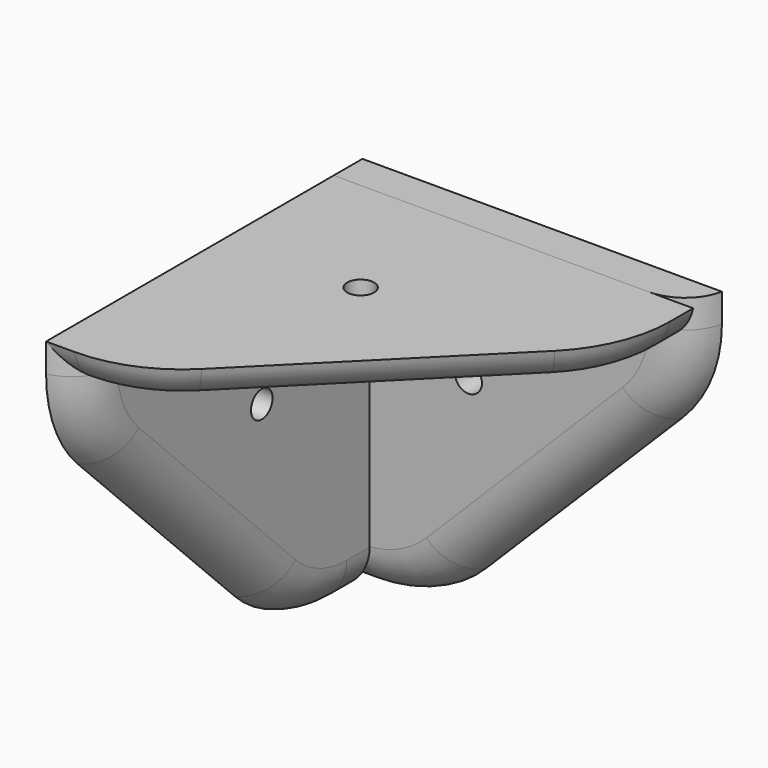
from build123d import *

# Parameters (mm, degrees)
F0_R           = 1.5
F1_DEPTH       = 4
F2_R           = 15
F3_ANGLE       = 90
F4_ANGLE       = 270
F5_T1_DEPTH    = 30.8664248821
F5_T3_DEPTH    = 15.4215903688
F5_T5_DEPTH    = 15.4215903688
F5_T8_ANGLE    = 45
F5_T10_ANGLE   = 45
F5_2_T1_DEPTH  = 30.8664248821
F5_2_T3_DEPTH  = 15.4215903688
F5_2_T5_DEPTH  = 15.4215903688
F5_2_T8_ANGLE  = 45
F5_2_T10_ANGLE = 45
F5_3_T1_DEPTH  = 30.8664248821
F5_3_T3_DEPTH  = 15.4215903688
F5_3_T5_DEPTH  = 15.4215903688
F5_3_T8_ANGLE  = 45
F5_3_T10_ANGLE = 45


# Not quite as in the source:
# - a fillet or chamfer that OpenCascade refuses, or shapes differently, is made with other operations: its cross-section is extruded or revolved along the edge and cut away or added


with BuildPart() as f1:
    # F0 (on Front) → F1 (new body)
    with BuildSketch(Plane.XZ):
        Polygon((40, 0), (0, 0), (0, -40), (9.3873450905, -40), (40, -9.3873450905), align=None)
        with Locations((15, -15)):
            Circle(F0_R, mode=Mode.SUBTRACT)
    extrude(amount=-F1_DEPTH)

    # F2
    f2_edges = [f1.edges().sort_by_distance(p)[0] for p in [
        (9.387345, 2, -40),
        (40, 2, -9.387345),
    ]]
    fillet(f2_edges, radius=F2_R)


with BuildPart() as f3_1:
    # F3: copy of F1
    add(f1.part.rotate(Axis((0, 0, -20), (0, 0, -1)), F3_ANGLE))

    # F5#2: fillet of radius 5 on 1 edges, made by hand

    # F5_2_s2 → F5_2_t1 (cut)
    with BuildSketch(Plane(origin=(0, 10.9129291725, -10.9129291725), x_dir=(1, 0, 0), z_dir=(0, -0.7071067812, 0.7071067812))):
        with BuildLine():
            ThreePointArc((0, -34.9221266183), (2.8729833462, -33.1854247929), (4, -30.0231471327))
            Line((4, -30.0231471327), (4, -34.9221266183))
            Line((4, -34.9221266183), (0, -34.9221266183))
        make_face()
    extrude(amount=F5_2_T1_DEPTH, mode=Mode.SUBTRACT)

    # F5_2_s4 → F5_2_t3 (cut)
    with BuildSketch(Plane.XY.offset(-3.1741416549)):
        with BuildLine():
            ThreePointArc((4, -35.1010205144), (2.8729833462, -38.2632981746), (0, -40))
            Line((0, -40), (4, -40))
            Line((4, -40), (4, -35.1010205144))
        make_face()
    extrude(amount=F5_2_T3_DEPTH, mode=Mode.SUBTRACT)

    # F5_2_s6 → F5_2_t5 (cut)
    with BuildSketch(Plane.XZ.offset(-12.2474487139)):
        with BuildLine():
            ThreePointArc((4, -35.1010205144), (2.8729833462, -38.2632981746), (0, -40))
            Line((0, -40), (4, -40))
            Line((4, -40), (4, -35.1010205144))
        make_face()
    extrude(amount=F5_2_T5_DEPTH, mode=Mode.SUBTRACT)

    # F5_2_s7 → F5_2_t8 (revolve, cut)
    with BuildSketch(Plane(origin=(0, 10.9129291725, -10.9129291725), x_dir=(1, 0, 0), z_dir=(0, -0.7071067812, 0.7071067812))):
        with BuildLine():
            ThreePointArc((0, -34.9221266183), (2.8729833462, -33.1854247929), (4, -30.0231471327))
            Line((4, -30.0231471327), (4, -34.9221266183))
            Line((4, -34.9221266183), (0, -34.9221266183))
        make_face()
    revolve(axis=Axis((4, -3.1741416549, -25), (1, 0, 0)), revolution_arc=F5_2_T8_ANGLE, mode=Mode.SUBTRACT)

    # F5_2_s9 → F5_2_t10 (revolve, cut)
    with BuildSketch(Plane(origin=(0, -10.9129291725, 10.9129291725), x_dir=(1, 0, 0), z_dir=(0, 0.7071067812, -0.7071067812))):
        with BuildLine():
            ThreePointArc((0, 34.9221266183), (2.8729833462, 33.1854247929), (4, 30.0231471327))
            Line((4, 30.0231471327), (4, 34.9221266183))
            Line((4, 34.9221266183), (0, 34.9221266183))
        make_face()
    revolve(axis=Axis((4, -25, -3.1741416549), (-1, 0, 0)), revolution_arc=F5_2_T10_ANGLE, mode=Mode.SUBTRACT)


with BuildPart() as f4_1:
    # F4: copy of F1
    add(f1.part.rotate(Axis((20, 0, 0), (1, 0, 0)), F4_ANGLE))

    # F5#3: fillet of radius 5 on 1 edges, made by hand

    # F5_3_s2 → F5_3_t1 (cut)
    with BuildSketch(Plane(origin=(-10.9129291725, -10.9129291725, 0), x_dir=(0, 0, 1), z_dir=(0.7071067812, 0.7071067812, 0))):
        with BuildLine():
            ThreePointArc((0, 34.9221266183), (-2.8729833462, 33.1854247929), (-4, 30.0231471327))
            Line((-4, 30.0231471327), (-4, 34.9221266183))
            Line((-4, 34.9221266183), (0, 34.9221266183))
        make_face()
    extrude(amount=F5_3_T1_DEPTH, mode=Mode.SUBTRACT)

    # F5_3_s4 → F5_3_t3 (cut)
    with BuildSketch(Plane.XZ.offset(-12.2474487139)):
        with BuildLine():
            ThreePointArc((35.1010205144, -4), (38.2632981746, -2.8729833462), (40, 0))
            Line((40, 0), (40, -4))
            Line((40, -4), (35.1010205144, -4))
        make_face()
    extrude(amount=F5_3_T3_DEPTH, mode=Mode.SUBTRACT)

    # F5_3_s6 → F5_3_t5 (cut)
    with BuildSketch(Plane.YZ.offset(-12.2474487139)):
        with BuildLine():
            ThreePointArc((-35.1010205144, -4), (-38.2632981746, -2.8729833462), (-40, 0))
            Line((-40, 0), (-40, -4))
            Line((-40, -4), (-35.1010205144, -4))
        make_face()
    extrude(amount=F5_3_T5_DEPTH, mode=Mode.SUBTRACT)

    # F5_3_s7 → F5_3_t8 (revolve, cut)
    with BuildSketch(Plane(origin=(-10.9129291725, -10.9129291725, 0), x_dir=(0, 0, 1), z_dir=(0.7071067812, 0.7071067812, 0))):
        with BuildLine():
            ThreePointArc((0, 34.9221266183), (-2.8729833462, 33.1854247929), (-4, 30.0231471327))
            Line((-4, 30.0231471327), (-4, 34.9221266183))
            Line((-4, 34.9221266183), (0, 34.9221266183))
        make_face()
    revolve(axis=Axis((3.1741416549, -25, -4), (0, 0, -1)), revolution_arc=F5_3_T8_ANGLE, mode=Mode.SUBTRACT)

    # F5_3_s9 → F5_3_t10 (revolve, cut)
    with BuildSketch(Plane(origin=(10.9129291725, 10.9129291725, 0), x_dir=(0, 0, 1), z_dir=(-0.7071067812, -0.7071067812, 0))):
        with BuildLine():
            ThreePointArc((0, -34.9221266183), (-2.8729833462, -33.1854247929), (-4, -30.0231471327))
            Line((-4, -30.0231471327), (-4, -34.9221266183))
            Line((-4, -34.9221266183), (0, -34.9221266183))
        make_face()
    revolve(axis=Axis((25, -3.1741416549, -4), (0, 0, 1)), revolution_arc=F5_3_T10_ANGLE, mode=Mode.SUBTRACT)


with BuildPart() as f1_1:
    add(f1.part)

    # F5: fillet of radius 5 on 1 edges, made by hand

    # F5_s2 → F5_t1 (cut)
    with BuildSketch(Plane(origin=(-10.9129291725, 0, -10.9129291725), x_dir=(0, 1, 0), z_dir=(0.7071067812, 0, 0.7071067812))):
        with BuildLine():
            ThreePointArc((4, -34.9221266183), (1.1270166538, -33.1854247929), (0, -30.0231471327))
            Line((0, -30.0231471327), (0, -34.9221266183))
            Line((0, -34.9221266183), (4, -34.9221266183))
        make_face()
    extrude(amount=F5_T1_DEPTH, mode=Mode.SUBTRACT)

    # F5_s4 → F5_t3 (cut)
    with BuildSketch(Plane.XY.offset(-3.1741416549)):
        with BuildLine():
            ThreePointArc((35.1010205144, 0), (38.2632981746, 1.1270166538), (40, 4))
            Line((40, 4), (40, 0))
            Line((40, 0), (35.1010205144, 0))
        make_face()
    extrude(amount=F5_T3_DEPTH, mode=Mode.SUBTRACT)

    # F5_s6 → F5_t5 (cut)
    with BuildSketch(Plane.YZ.offset(-12.2474487139)):
        with BuildLine():
            ThreePointArc((0, -35.1010205144), (1.1270166538, -38.2632981746), (4, -40))
            Line((4, -40), (0, -40))
            Line((0, -40), (0, -35.1010205144))
        make_face()
    extrude(amount=F5_T5_DEPTH, mode=Mode.SUBTRACT)

    # F5_s7 → F5_t8 (revolve, cut)
    with BuildSketch(Plane(origin=(-10.9129291725, 0, -10.9129291725), x_dir=(0, 1, 0), z_dir=(0.7071067812, 0, 0.7071067812))):
        with BuildLine():
            ThreePointArc((0, -30.0231471327), (1.1270166538, -33.1854247929), (4, -34.9221266183))
            Line((4, -34.9221266183), (0, -34.9221266183))
            Line((0, -34.9221266183), (0, -30.0231471327))
        make_face()
    revolve(axis=Axis((3.1741416549, 0, -25), (0, 1, 0)), revolution_arc=F5_T8_ANGLE, mode=Mode.SUBTRACT)

    # F5_s9 → F5_t10 (revolve, cut)
    with BuildSketch(Plane(origin=(10.9129291725, 0, 10.9129291725), x_dir=(0, 1, 0), z_dir=(-0.7071067812, 0, -0.7071067812))):
        with BuildLine():
            ThreePointArc((0, 30.0231471327), (1.1270166538, 33.1854247929), (4, 34.9221266183))
            Line((4, 34.9221266183), (0, 34.9221266183))
            Line((0, 34.9221266183), (0, 30.0231471327))
        make_face()
    revolve(axis=Axis((25, 0, -3.1741416549), (0, -1, 0)), revolution_arc=F5_T10_ANGLE, mode=Mode.SUBTRACT)


solid = Compound([f3_1.part, f4_1.part, f1_1.part])
